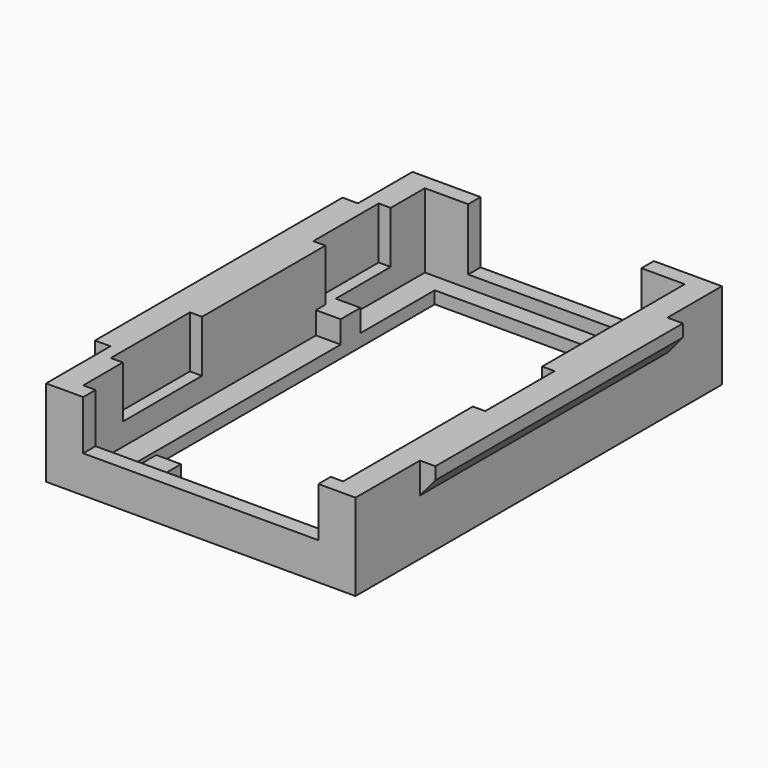
from build123d import *

# Parameters (mm, degrees)
F0_W      = 25
F0_H      = 38
F1_DEPTH  = 7
F2_W      = 21
F2_H      = 34.5
F3_DEPTH  = 6
F4_W      = 2
F4_H      = 2
F5_DEPTH  = 1.8
F6_W      = 17
F6_H      = 31.25
F7_DEPTH  = 7.001
F8_W      = 0.0254269466
F8_H      = 6.6
F8_W_2    = 0.9745730534
F8_W_3    = 1
F8_H_2    = 7
F8_H_3    = 8
F9_DEPTH  = 4.2
F11_W     = 14
F11_H     = 5
F12_DEPTH = 5
F13_DEPTH = 1
F15_DEPTH = 12.5
F16_W     = 19
F16_H     = 4
F17_DEPTH = 3


# Not quite as in the source:
# - a pattern or mirror of a feature is missing from the dataset's text; its kind, count and spacing are read off the source's solid
# - a feature names something its author has since deleted; it is built from what else it names


with BuildPart() as f1:
    # F0 (on Top) → F1 (new body)
    with BuildSketch(Plane.XY):
        Rectangle(F0_W, F0_H)
    extrude(amount=F1_DEPTH)

    # F2 (on face) → F3 (cut)
    with BuildSketch(Plane.XY.offset(7)):
        with Locations((0, -0.5)):
            Rectangle(F2_W, F2_H)
    extrude(amount=-F3_DEPTH, mode=Mode.SUBTRACT)

    # F4 (on face) → F5 (join)
    with BuildSketch(Plane.XY.offset(1)):
        with Locations((-9.5, 6.75)):
            Rectangle(F4_W, F4_H)
        with Locations((9.5, 6.75)):
            Rectangle(F4_W, F4_H)
        with Locations((9.5, -9.75)):
            Rectangle(F4_W, F4_H)
        with Locations((-5, -17)):
            Rectangle(F4_W, F4_H)
    extrude(amount=F5_DEPTH)

    # F6 (on Top) → F7 (cut, through all)
    with BuildSketch(Plane.XY):
        with Locations((0, -0.375)):
            Rectangle(F6_W, F6_H)
    extrude(amount=F7_DEPTH, mode=Mode.SUBTRACT)

    # F8 (on face) → F9 (cut, through all)
    with BuildSketch(Plane.XY.offset(7)):
        with Locations((-10.4872865267, 10.0065428064)):
            Rectangle(F8_W, F8_H)
        with Locations((-10.9872865267, 10.0065428064)):
            Rectangle(F8_W_2, F8_H)
        with Locations((11, -1.15)):
            Rectangle(F8_W_3, F8_H_2)
        with Locations((-10.9872865267, -9.75)):
            Rectangle(F8_W_2, F8_H_3)
    extrude(amount=-F9_DEPTH, mode=Mode.SUBTRACT)

    # F11 (on offset) → F12 (cut)
    with BuildSketch(Plane.XY.offset(2)):
        with Locations((0, 19.25)):
            Rectangle(F11_W, F11_H)
    extrude(amount=F12_DEPTH, mode=Mode.SUBTRACT)

    # F13 (cut): a face of the model
    f13_faces = [f1.faces().sort_by_distance(p)[0] for p in [
        (0, 19, 0.2596150997),
    ]]
    extrude(f13_faces, amount=-F13_DEPTH, mode=Mode.SUBTRACT)

    # F14 (on Front) → F15 (join, symmetric)
    with BuildSketch(Plane.XZ):
        Polygon((13.75, 7), (12.5, 7), (12.5, 4.5103080093), (13.75, 6), align=None)
    f15 = extrude(amount=F15_DEPTH, both=True)

    # F15_copies: F15 across plane
    add(f15.mirror(Plane(origin=(0, 0, 0), x_dir=(0, 0, -1), z_dir=(-1, 0, 0))))

    # F16 (on face) → F17 (cut)
    with BuildSketch(Plane.XZ.offset(19)):
        with Locations((0, 5)):
            Rectangle(F16_W, F16_H)
    extrude(amount=-F17_DEPTH, mode=Mode.SUBTRACT)


solid = f1.part
